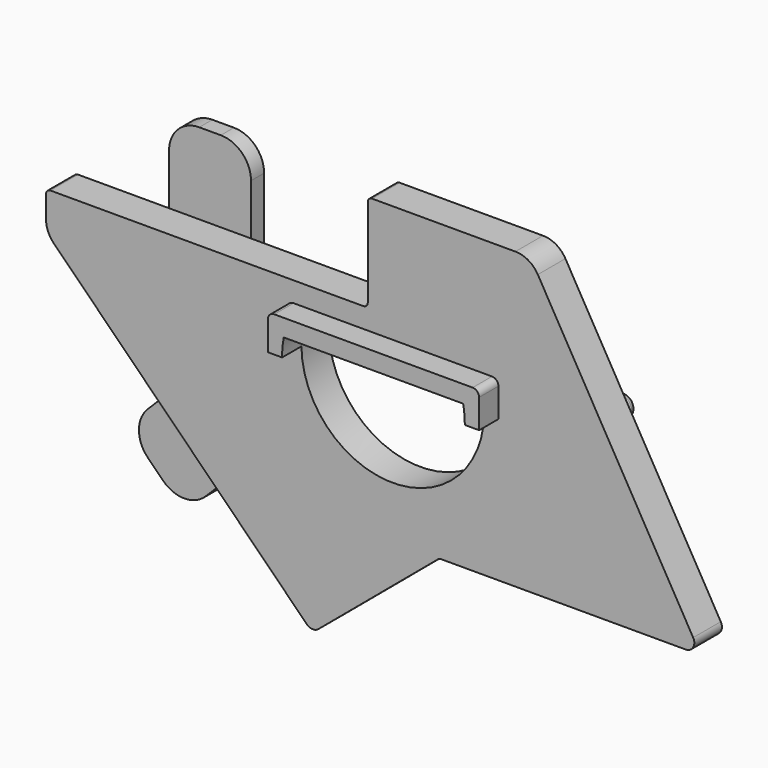
from build123d import *
from build123d import SkipClean  # not in build123d's __all__

# Parameters (mm, degrees)
F1_DEPTH  = 4
F2_R      = 3
F3_R      = 1
F4_R      = 0.5
F6_DEPTH  = 25
F8_DEPTH  = 2.8
F9_R      = 0.75
F10_W     = 9.5
F10_H     = 9.4
F10_H_2   = 5.1
F11_DEPTH = 1.9
F12_R     = 3.5
F13_R     = 1.325
F14_DEPTH = 5
F15_R     = 0.7


# Not quite as in the source:
# - after a boolean that leaves OpenCascade's solid faulty, fix() repairs it


with BuildPart() as f1:
    # F0 (on Front) → F1 (new body)
    with BuildSketch(Plane.XZ):
        Polygon((0, 11.3), (0, 0), (-37.3, 0), (-37.3, -4.37), (-6.42, -35.25), (8.2981568685, -22.9), (38.5981568685, -22.9), (18.8527776623, 11.3), align=None)
    extrude(amount=F1_DEPTH)

    # F2
    f2_edges = [f1.edges().sort_by_distance(p)[0] for p in [
        (-37.3, -2, -4.37),
        (18.852778, -2, 11.3),
    ]]
    fillet(f2_edges, radius=F2_R)

    # F3
    f3_edges = [f1.edges().sort_by_distance(p)[0] for p in [
        (38.598157, -2, -22.9),
        (-6.42, -2, -35.25),
    ]]
    fillet(f3_edges, radius=F3_R)

    # F4
    f4_edges = [f1.edges().sort_by_distance(p)[0] for p in [
        (8.298157, -2, -22.9),
        (0, -2, 0),
        (0, -2, 11.3),
        (-37.3, -2, 0),
    ]]
    fillet(f4_edges, radius=F4_R)

    # F5 (on face) → F6 (cut)
    with BuildSketch(Plane.XZ.offset(4)):
        with BuildLine():
            Line((13.3, -4.33), (-7.5, -4.33))
            ThreePointArc((-7.5, -4.33), (2.9, -16.93), (13.3, -4.33))
        make_face()
    extrude(amount=-F6_DEPTH, mode=Mode.SUBTRACT)

    # F7 (on face) → F8 (join)
    with BuildSketch(Plane.XZ.offset(4)):
        with BuildLine():
            Line((15.15, -2.33), (-9.35, -2.33))
            Line((-9.35, -2.33), (-9.35, -6.44))
            Line((-9.35, -6.44), (-7.6915717466, -6.44))
            ThreePointArc((-7.6915717466, -6.44), (-7.6486750873, -5.3801980668), (-7.5, -4.33))
            Line((-7.5, -4.33), (13.3, -4.33))
            ThreePointArc((13.3, -4.33), (13.4486750873, -5.3801980668), (13.4915717466, -6.44))
            Line((13.4915717466, -6.44), (15.15, -6.44))
            Line((15.15, -6.44), (15.15, -2.33))
        make_face()
    with SkipClean():  # cleaning this boolean's faces spoils the solid; the shape is the same uncleaned
        extrude(amount=F8_DEPTH)

    # F9
    f9_edges = [f1.edges().sort_by_distance(p)[0] for p in [
        (-9.35, -5.4, -2.33),
        (15.15, -5.4, -2.33),
    ]]
    fillet(f9_edges, radius=F9_R)

    # F10 (on face) → F11 (join)
    with BuildSketch(Plane(origin=(0, 0, 0), x_dir=(-1, 0, 0), z_dir=(0, 1, 0))):
        with Locations((21.49, 4.7)):
            Rectangle(F10_W, F10_H)
        with Locations((21.49, -2.55)):
            Rectangle(F10_W, F10_H_2)
        Polygon((17.8186578158, -23.8513421842), (24.5361722371, -17.1338277629), (20.929927653, -13.5275831789), (14.2124132317, -20.2450976002), align=None)
        Polygon((31.1829759802, -23.7806315061), (24.5361722371, -17.1338277629), (17.8186578158, -23.8513421842), (24.4654615589, -30.4981459274), align=None)
    extrude(amount=F11_DEPTH)

    add(f1.part.fix(), mode=Mode.REPLACE)

    # F12
    f12_edges = [f1.edges().sort_by_distance(p)[0] for p in [
        (-24.465462, 0.95, -30.498146),
        (-31.182976, 0.95, -23.780632),
        (-14.212413, 0.95, -20.245098),
        (-20.929928, 0.95, -13.527583),
        (-26.24, 0.95, 9.4),
        (-16.74, 0.95, 9.4),
        (-26.24, 0.95, -5.1),
        (-16.74, 0.95, -5.1),
    ]]
    fillet(f12_edges, radius=F12_R)

    # F13 (on face) → F14 (join)
    with BuildSketch(Plane(origin=(0, 0, 0), x_dir=(-1, 0, 0), z_dir=(0, 1, 0))):
        with Locations((-22.6430821795, -6.115)):
            Circle(F13_R)
    extrude(amount=F14_DEPTH)

    # F15
    f15_edges = [f1.edges().sort_by_distance(p)[0] for p in [
        (23.968082, 5, -6.115),
    ]]
    fillet(f15_edges, radius=F15_R)


solid = f1.part
